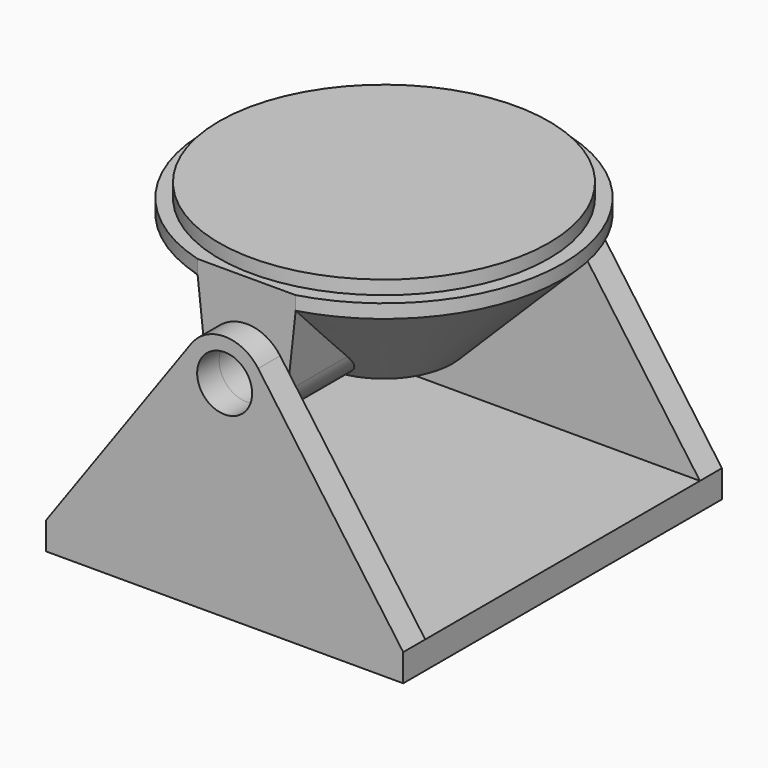
from build123d import *

# Parameters (mm, degrees)
F0_W      = 330.2
F0_H      = 317.5
F1_DEPTH  = 25.4
F2_W      = 330.2
F2_H      = 25.4
F2_R      = 25.4
F3_DEPTH  = 25.4
F7_DEPTH  = 12.7
F7_FACE_R = 165.1
F8_DEPTH  = 101.6
F8_TAPER  = 45
F9_DEPTH  = 266.701
F10_R     = 25.4
F11_DEPTH = 317.5
F12_R     = 152.4
F13_DEPTH = 12.7


with BuildPart() as f1:
    # F0 (on Top) → F1 (new body)
    with BuildSketch(Plane.XY):
        Rectangle(F0_W, F0_H)
    extrude(amount=F1_DEPTH)

    # F2 (on face) → F3 (join)
    with BuildSketch(Plane.XZ.offset(158.75)):
        with Locations((0, 12.7)):
            Rectangle(F2_W, F2_H)
        with BuildLine():
            Line((-30.975823358, 212.6835156657), (-165.1, 25.4))
            Line((-165.1, 25.4), (165.1, 25.4))
            Line((165.1, 25.4), (30.975823358, 212.6835156657))
            ThreePointArc((30.975823358, 212.6835156657), (36.2752592681, 202.149702358), (38.1, 190.5))
            ThreePointArc((38.1, 190.5), (-11.649702358, 154.2247407319), (-30.975823358, 212.6835156657))
        make_face()
        with BuildLine():
            ThreePointArc((30.975823358, 212.6835156657), (0, 228.6), (-30.975823358, 212.6835156657))
            ThreePointArc((-30.975823358, 212.6835156657), (-11.649702358, 154.2247407319), (38.1, 190.5))
            ThreePointArc((38.1, 190.5), (36.2752592681, 202.149702358), (30.975823358, 212.6835156657))
        make_face()
        with Locations((0, 190.5)):
            Circle(F2_R, mode=Mode.SUBTRACT)
    extrude(amount=F3_DEPTH)

    # F4: F1 across plane


with BuildPart() as f1_1:
    add(f1.part)
    add(f1.part.mirror(Plane.XZ))


with BuildPart() as f7:
    # F6 (on offset) → F7 (new body)
    with BuildSketch(Plane.XY.offset(266.7)):
        with BuildLine():
            ThreePointArc((45.3480705212, -158.75), (131.8047352015, -99.4259612902), (165.1, 0))
            ThreePointArc((165.1, 0), (131.8047352015, 99.4259612902), (45.3480705212, 158.75))
            Line((45.3480705212, 158.75), (-45.3480705212, 158.75))
            ThreePointArc((-45.3480705212, 158.75), (-165.1, 0), (-45.3480705212, -158.75))
            Line((-45.3480705212, -158.75), (45.3480705212, -158.75))
        make_face()
        with BuildLine():
            ThreePointArc((-45.3480705212, -158.75), (0, -165.1), (45.3480705212, -158.75))
            Line((45.3480705212, -158.75), (-45.3480705212, -158.75))
        make_face()
        with BuildLine():
            Line((-45.3480705212, 158.75), (45.3480705212, 158.75))
            ThreePointArc((45.3480705212, 158.75), (0, 165.1), (-45.3480705212, 158.75))
        make_face()
    extrude(amount=-F7_DEPTH)

    # F7_face (on face) → F8 (join)
    with BuildSketch(Plane(origin=(0, 0, 254), x_dir=(1, 0, 0), z_dir=(0, 0, -1))):
        Circle(F7_FACE_R)
    extrude(amount=F8_DEPTH, taper=F8_TAPER)

    # F6 (on offset) → F9 (cut, through all)
    with BuildSketch(Plane.XY.offset(266.7)):
        with BuildLine():
            Line((-45.3480705212, 158.75), (45.3480705212, 158.75))
            ThreePointArc((45.3480705212, 158.75), (0, 165.1), (-45.3480705212, 158.75))
        make_face()
        with BuildLine():
            ThreePointArc((-45.3480705212, -158.75), (0, -165.1), (45.3480705212, -158.75))
            Line((45.3480705212, -158.75), (-45.3480705212, -158.75))
        make_face()
    extrude(amount=-F9_DEPTH, mode=Mode.SUBTRACT)

    # F10 (on face) → F11 (join, through all)
    with BuildSketch(Plane.XZ.offset(158.75)):
        with BuildLine():
            ThreePointArc((38.1, 190.5), (-2.0953009818, 228.5423410662), (-37.8695387819, 186.3157399167))
            ThreePointArc((-37.8695387819, 186.3157399167), (0, 152.4), (37.8695387819, 186.3157399167))
            ThreePointArc((37.8695387819, 186.3157399167), (38.0423410662, 188.4046990182), (38.1, 190.5))
        make_face()
        with Locations((0, 190.5)):
            Circle(F10_R, mode=Mode.SUBTRACT)
        with BuildLine():
            add(Edge.make_bspline(
                [(-45.3480705212, 254), (0, 241.5442307692), (45.3480705212, 254)],
                knots=[-0.2819082891, -0.2819082891, -0.2819082891, 0.2819082891, 0.2819082891, 0.2819082891], degree=2, weights=[1, 1.04, 1]))
            Line((-45.3480705212, 254), (-37.8695387819, 186.3157399167))
            ThreePointArc((-37.8695387819, 186.3157399167), (-2.0953009818, 228.5423410662), (38.1, 190.5))
            ThreePointArc((38.1, 190.5), (38.0423410662, 188.4046990182), (37.8695387819, 186.3157399167))
            Line((37.8695387819, 186.3157399167), (45.3480705212, 254))
        make_face()
    extrude(amount=-F11_DEPTH)


with BuildPart() as f13:
    # F12 (on face) → F13 (new body)
    with BuildSketch(Plane.XY.offset(266.7)):
        Circle(F12_R)
    extrude(amount=F13_DEPTH)


solid = Compound([f1_1.part, f7.part, f13.part])
